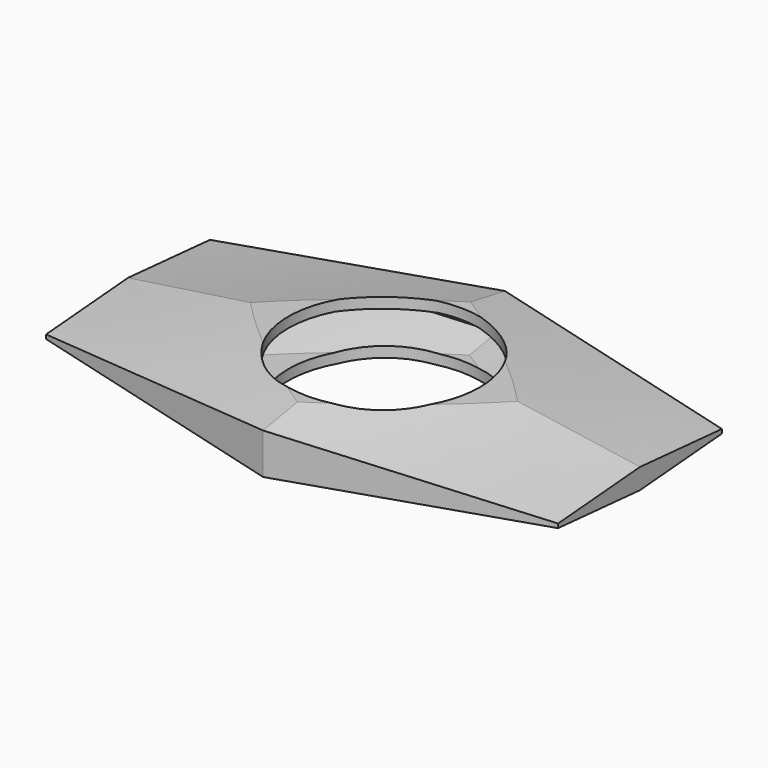
from build123d import *

# Parameters (mm, degrees)
F7_R      = 11.88
F8_DEPTH  = 12.7
F9_W      = 64.8597117375
F9_H      = 17.9217835129
F9_W_2    = 54.5544467036
F9_H_2    = 7
F10_DEPTH = 38.1
F11_T     = 1.27


# Not quite as in the source:
# - a shell that OpenCascade refuses in one call is made with other operations: the cavity is built on its own and cut out


with BuildPart() as f3:
    # F0 (on Right) → F3 section 0
    with BuildSketch(Plane.YZ):
        Polygon((-18.738, 2.54), (-18.738, 0), (-18.738, -2.54), (0, -5.9280314961), (18.738, -2.54), (18.738, 0), (18.738, 2.54), (0, 5.9280314961), align=None)
    # F2 (on offset) → F3 section 1
    with BuildSketch(Plane.YZ.offset(31.75)):
        Polygon((-12.7, 0.254), (-12.7, 0), (-12.7, -0.254), (0, -1.27), (12.7, -0.254), (12.7, 0), (12.7, 0.254), (0, 1.27), align=None)
    loft()

    # F0 (on Right) → F6 section 0
    with BuildSketch(Plane.YZ):
        Polygon((-18.738, 2.54), (-18.738, 0), (-18.738, -2.54), (0, -5.9280314961), (18.738, -2.54), (18.738, 0), (18.738, 2.54), (0, 5.9280314961), align=None)
    # F5 (on offset) → F6 section 1
    with BuildSketch(Plane.YZ.offset(-31.75)):
        Polygon((-12.7, 0.254), (-12.7, 0), (-12.7, -0.254), (0, -1.27), (12.7, -0.254), (12.7, 0), (12.7, 0.254), (0, 1.27), align=None)
    loft()

    # F7 (on Top) → F8 (cut, symmetric)
    with BuildSketch(Plane.XY):
        Circle(F7_R)
    extrude(amount=F8_DEPTH, both=True, mode=Mode.SUBTRACT)

    # F9 (on Right) → F10 (cut, symmetric)
    with BuildSketch(Plane.YZ):
        Rectangle(F9_W, F9_H)
        Rectangle(F9_W_2, F9_H_2, mode=Mode.SUBTRACT)
    extrude(amount=F10_DEPTH, both=True, mode=Mode.SUBTRACT)

    # F11: shell of thickness 1.27, made by hand


with BuildPart() as f11_core1:
    # F11_t2: copy of F3
    add(f3.part)

    # the walls: a layer under each face that stays
    f11_faces = [f11_core1.faces().sort_by_distance(p)[0] for p in [
        (15.815318863, -15.7303497545, -0.570701626),
        (-15.815318863, -15.7303497545, -0.570701626),
        (15.875, -7.8595, -2.498007874),
        (31.75, 0, 0),
        (15.875, -7.8595, 2.498007874),
        (-15.875, -7.8595, -2.498007874),
        (-31.75, 0, 0),
        (-15.875, -7.8595, 2.498007874),
        (15.875, 7.8595, -2.498007874),
        (13.44910738, 0, -3.5),
        (0, -12.4848744889, -3.5),
        (15.815318863, 15.7303497545, 0.570701626),
        (15.875, 7.8595, 2.498007874),
        (13.44910738, 0, 3.5),
        (0, -12.4848744889, 3.5),
        (-15.875, 7.8595, -2.498007874),
        (-13.44910738, 0, -3.5),
        (-15.815318863, 15.7303497545, 0.570701626),
        (-15.875, 7.8595, 2.498007874),
        (-13.44910738, 0, 3.5),
        (0, 12.4848744889, -3.5),
        (0, 12.4848744889, 3.5),
    ]]
    thicken(f11_faces, amount=-F11_T, mode=Mode.SUBTRACT)


with BuildPart() as f3_1:
    add(f3.part)

    # what is left inside the walls is the cavity
    f11_cavity = [f11_core1.part.solids().sort_by_distance(p)[0] for p in [
        (-11.8927, 0, -0.743333),
    ]]
    add(f11_cavity, mode=Mode.SUBTRACT)


solid = f3_1.part
